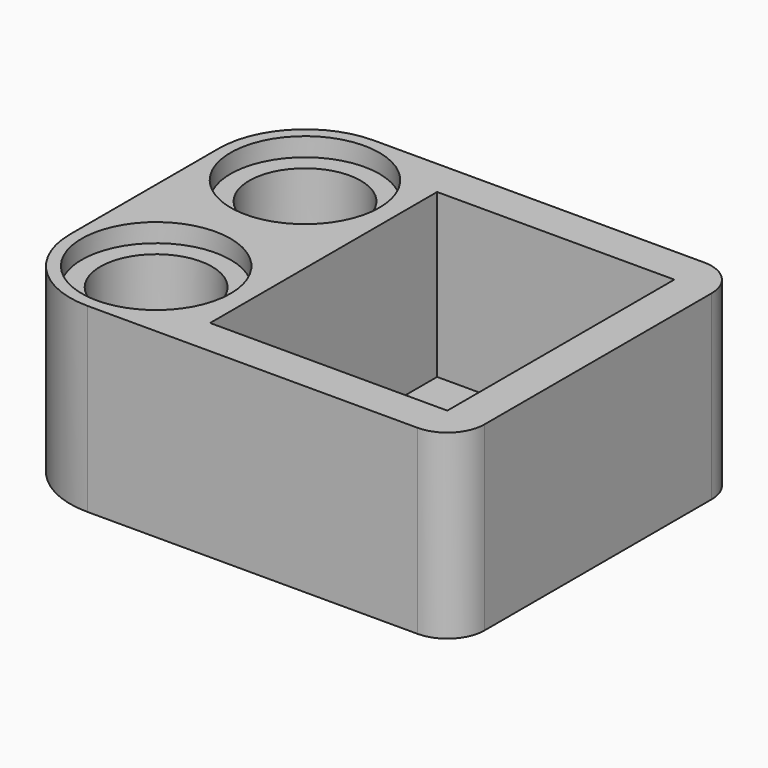
from build123d import *

# Parameters (mm, degrees)
F0_R     = 3.2
F0_W     = 10.2
F0_H     = 12.2
F1_DEPTH = 7.8
F2_START = 0.8
F0_R_2   = 2.4
F2_DEPTH = 6.2
F0_R_3   = 1
F0_R_4   = 2
F3_DEPTH = 0.8


# Not quite as in the source:
# - a feature names something its author has since deleted; it is built from what else it names


with BuildPart() as f1:
    # F0 (on Top) → F1 (new body)
    with BuildSketch(Plane.XY):
        with BuildLine():
            Line((5.1, 7.7), (-9.1, 7.7))
            ThreePointArc((-9.1, 7.7), (-11.7162950904, 6.6162950904), (-12.8, 4))
            Line((-12.8, 4), (-12.8, -4))
            ThreePointArc((-12.8, -4), (-11.7162950904, -6.6162950904), (-9.1, -7.7))
            Line((-9.1, -7.7), (5.1, -7.7))
            ThreePointArc((5.1, -7.7), (6.2313708499, -7.2313708499), (6.7, -6.1))
            Line((6.7, -6.1), (6.7, 6.1))
            ThreePointArc((6.7, 6.1), (6.2313708499, 7.2313708499), (5.1, 7.7))
        make_face()
        with Locations((-9.1, -4)):
            Circle(F0_R, mode=Mode.SUBTRACT)
        with Locations((-9.1, 4)):
            Circle(F0_R, mode=Mode.SUBTRACT)
        Rectangle(F0_W, F0_H, mode=Mode.SUBTRACT)
    extrude(amount=F1_DEPTH)

    # F0 (on Top) → F2 (join)
    with BuildSketch(Plane.XY.offset(F2_START)):
        with Locations((-9.1, -4)):
            Circle(F0_R)
        with Locations((-9.1, -4)):
            Circle(F0_R_2, mode=Mode.SUBTRACT)
        with Locations((-9.1, 4)):
            Circle(F0_R)
        with Locations((-9.1, 4)):
            Circle(F0_R_2, mode=Mode.SUBTRACT)
    extrude(amount=F2_DEPTH)

    # F0 (on Top) → F3 (join)
    with BuildSketch(Plane.XY):
        Rectangle(F0_W, F0_H)
        with Locations((0, -4.5)):
            Circle(F0_R_3, mode=Mode.SUBTRACT)
        Circle(F0_R_4, mode=Mode.SUBTRACT)
        with Locations((0, 4.5)):
            Circle(F0_R_3, mode=Mode.SUBTRACT)
    extrude(amount=F3_DEPTH)


solid = f1.part
